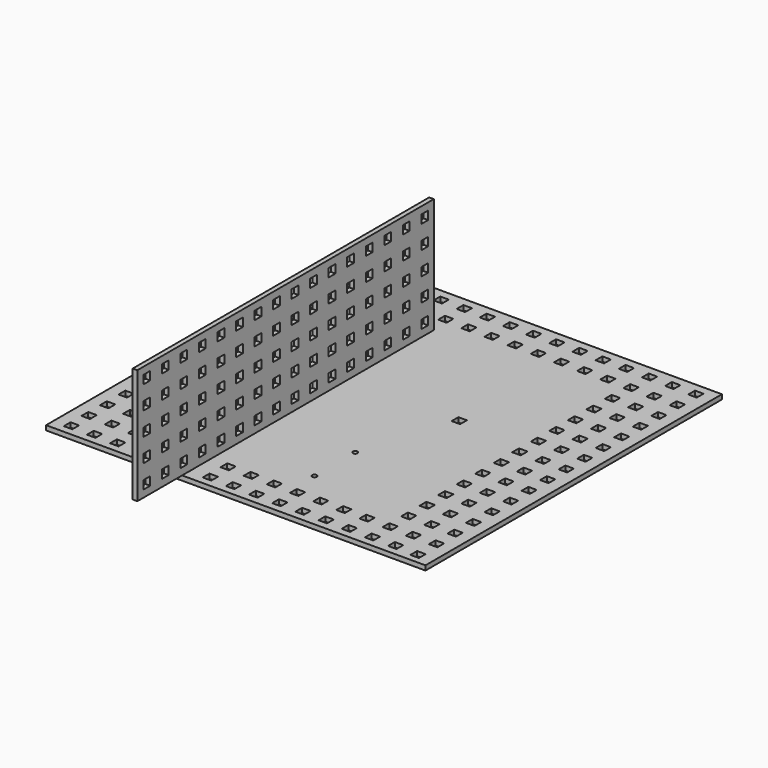
from build123d import *

# Parameters (mm, degrees)
F1_W     = 203.2
F1_H     = 63.246
F1_W_2   = 4.6228
F1_H_2   = 4.6228
F2_DEPTH = 2.54
F0_W     = 4.6482
F0_H     = 4.6228
F0_W_2   = 4.6228
F0_H_2   = 4.6482
F0_R     = 1.27
F3_DEPTH = 2.54


# Not quite as in the source:
# - a feature names something its author has since deleted; it is built from what else it names


with BuildPart() as f2:
    # F1 (on Right) → F2 (new body)
    with BuildSketch(Plane.YZ):
        with Locations((9.3608458528, 31.623)):
            Rectangle(F1_W, F1_H)
        with Locations((-85.7621541472, 6.223)):
            Rectangle(F1_W_2, F1_H_2, mode=Mode.SUBTRACT)
        with Locations((-73.0621541472, 6.223)):
            Rectangle(F1_W_2, F1_H_2, mode=Mode.SUBTRACT)
        with Locations((-60.3621541472, 6.223)):
            Rectangle(F1_W_2, F1_H_2, mode=Mode.SUBTRACT)
        with Locations((-47.6621541472, 6.223)):
            Rectangle(F1_W_2, F1_H_2, mode=Mode.SUBTRACT)
        with Locations((-34.9621541472, 6.223)):
            Rectangle(F1_W_2, F1_H_2, mode=Mode.SUBTRACT)
        with Locations((-22.2621541472, 6.223)):
            Rectangle(F1_W_2, F1_H_2, mode=Mode.SUBTRACT)
        with Locations((-9.5621541472, 6.223)):
            Rectangle(F1_W_2, F1_H_2, mode=Mode.SUBTRACT)
        with Locations((3.1378458528, 6.223)):
            Rectangle(F1_W_2, F1_H_2, mode=Mode.SUBTRACT)
        with Locations((-85.7621541472, 18.923)):
            Rectangle(F1_W_2, F1_H_2, mode=Mode.SUBTRACT)
        with Locations((-73.0621541472, 18.923)):
            Rectangle(F1_W_2, F1_H_2, mode=Mode.SUBTRACT)
        with Locations((-60.3621541472, 18.923)):
            Rectangle(F1_W_2, F1_H_2, mode=Mode.SUBTRACT)
        with Locations((-47.6621541472, 18.923)):
            Rectangle(F1_W_2, F1_H_2, mode=Mode.SUBTRACT)
        with Locations((-85.7621541472, 31.623)):
            Rectangle(F1_W_2, F1_H_2, mode=Mode.SUBTRACT)
        with Locations((-73.0621541472, 31.623)):
            Rectangle(F1_W_2, F1_H_2, mode=Mode.SUBTRACT)
        with Locations((-60.3621541472, 31.623)):
            Rectangle(F1_W_2, F1_H_2, mode=Mode.SUBTRACT)
        with Locations((-47.6621541472, 31.623)):
            Rectangle(F1_W_2, F1_H_2, mode=Mode.SUBTRACT)
        with Locations((-34.9621541472, 18.923)):
            Rectangle(F1_W_2, F1_H_2, mode=Mode.SUBTRACT)
        with Locations((-22.2621541472, 18.923)):
            Rectangle(F1_W_2, F1_H_2, mode=Mode.SUBTRACT)
        with Locations((-9.5621541472, 18.923)):
            Rectangle(F1_W_2, F1_H_2, mode=Mode.SUBTRACT)
        with Locations((3.1378458528, 18.923)):
            Rectangle(F1_W_2, F1_H_2, mode=Mode.SUBTRACT)
        with Locations((-34.9621541472, 31.623)):
            Rectangle(F1_W_2, F1_H_2, mode=Mode.SUBTRACT)
        with Locations((-22.2621541472, 31.623)):
            Rectangle(F1_W_2, F1_H_2, mode=Mode.SUBTRACT)
        with Locations((-9.5621541472, 31.623)):
            Rectangle(F1_W_2, F1_H_2, mode=Mode.SUBTRACT)
        with Locations((3.1378458528, 31.623)):
            Rectangle(F1_W_2, F1_H_2, mode=Mode.SUBTRACT)
        with Locations((15.8378458528, 6.223)):
            Rectangle(F1_W_2, F1_H_2, mode=Mode.SUBTRACT)
        with Locations((28.5378458528, 6.223)):
            Rectangle(F1_W_2, F1_H_2, mode=Mode.SUBTRACT)
        with Locations((41.2378458528, 6.223)):
            Rectangle(F1_W_2, F1_H_2, mode=Mode.SUBTRACT)
        with Locations((53.9378458528, 6.223)):
            Rectangle(F1_W_2, F1_H_2, mode=Mode.SUBTRACT)
        with Locations((66.6378458528, 6.223)):
            Rectangle(F1_W_2, F1_H_2, mode=Mode.SUBTRACT)
        with Locations((79.3378458528, 6.223)):
            Rectangle(F1_W_2, F1_H_2, mode=Mode.SUBTRACT)
        with Locations((92.0378458528, 6.223)):
            Rectangle(F1_W_2, F1_H_2, mode=Mode.SUBTRACT)
        with Locations((104.7378458528, 6.223)):
            Rectangle(F1_W_2, F1_H_2, mode=Mode.SUBTRACT)
        with Locations((15.8378458528, 18.923)):
            Rectangle(F1_W_2, F1_H_2, mode=Mode.SUBTRACT)
        with Locations((28.5378458528, 18.923)):
            Rectangle(F1_W_2, F1_H_2, mode=Mode.SUBTRACT)
        with Locations((41.2378458528, 18.923)):
            Rectangle(F1_W_2, F1_H_2, mode=Mode.SUBTRACT)
        with Locations((53.9378458528, 18.923)):
            Rectangle(F1_W_2, F1_H_2, mode=Mode.SUBTRACT)
        with Locations((15.8378458528, 31.623)):
            Rectangle(F1_W_2, F1_H_2, mode=Mode.SUBTRACT)
        with Locations((28.5378458528, 31.623)):
            Rectangle(F1_W_2, F1_H_2, mode=Mode.SUBTRACT)
        with Locations((41.2378458528, 31.623)):
            Rectangle(F1_W_2, F1_H_2, mode=Mode.SUBTRACT)
        with Locations((53.9378458528, 31.623)):
            Rectangle(F1_W_2, F1_H_2, mode=Mode.SUBTRACT)
        with Locations((66.6378458528, 18.923)):
            Rectangle(F1_W_2, F1_H_2, mode=Mode.SUBTRACT)
        with Locations((79.3378458528, 18.923)):
            Rectangle(F1_W_2, F1_H_2, mode=Mode.SUBTRACT)
        with Locations((92.0378458528, 18.923)):
            Rectangle(F1_W_2, F1_H_2, mode=Mode.SUBTRACT)
        with Locations((104.7378458528, 18.923)):
            Rectangle(F1_W_2, F1_H_2, mode=Mode.SUBTRACT)
        with Locations((66.6378458528, 31.623)):
            Rectangle(F1_W_2, F1_H_2, mode=Mode.SUBTRACT)
        with Locations((79.3378458528, 31.623)):
            Rectangle(F1_W_2, F1_H_2, mode=Mode.SUBTRACT)
        with Locations((92.0378458528, 31.623)):
            Rectangle(F1_W_2, F1_H_2, mode=Mode.SUBTRACT)
        with Locations((104.7378458528, 31.623)):
            Rectangle(F1_W_2, F1_H_2, mode=Mode.SUBTRACT)
        with Locations((-85.7621541472, 44.323)):
            Rectangle(F1_W_2, F1_H_2, mode=Mode.SUBTRACT)
        with Locations((-73.0621541472, 44.323)):
            Rectangle(F1_W_2, F1_H_2, mode=Mode.SUBTRACT)
        with Locations((-60.3621541472, 44.323)):
            Rectangle(F1_W_2, F1_H_2, mode=Mode.SUBTRACT)
        with Locations((-47.6621541472, 44.323)):
            Rectangle(F1_W_2, F1_H_2, mode=Mode.SUBTRACT)
        with Locations((-34.9621541472, 44.323)):
            Rectangle(F1_W_2, F1_H_2, mode=Mode.SUBTRACT)
        with Locations((-22.2621541472, 44.323)):
            Rectangle(F1_W_2, F1_H_2, mode=Mode.SUBTRACT)
        with Locations((-9.5621541472, 44.323)):
            Rectangle(F1_W_2, F1_H_2, mode=Mode.SUBTRACT)
        with Locations((3.1378458528, 44.323)):
            Rectangle(F1_W_2, F1_H_2, mode=Mode.SUBTRACT)
        with Locations((-85.7621541472, 57.023)):
            Rectangle(F1_W_2, F1_H_2, mode=Mode.SUBTRACT)
        with Locations((-73.0621541472, 57.023)):
            Rectangle(F1_W_2, F1_H_2, mode=Mode.SUBTRACT)
        with Locations((-60.3621541472, 57.023)):
            Rectangle(F1_W_2, F1_H_2, mode=Mode.SUBTRACT)
        with Locations((-47.6621541472, 57.023)):
            Rectangle(F1_W_2, F1_H_2, mode=Mode.SUBTRACT)
        with Locations((-34.9621541472, 57.023)):
            Rectangle(F1_W_2, F1_H_2, mode=Mode.SUBTRACT)
        with Locations((-22.2621541472, 57.023)):
            Rectangle(F1_W_2, F1_H_2, mode=Mode.SUBTRACT)
        with Locations((-9.5621541472, 57.023)):
            Rectangle(F1_W_2, F1_H_2, mode=Mode.SUBTRACT)
        with Locations((3.1378458528, 57.023)):
            Rectangle(F1_W_2, F1_H_2, mode=Mode.SUBTRACT)
        with Locations((15.8378458528, 44.323)):
            Rectangle(F1_W_2, F1_H_2, mode=Mode.SUBTRACT)
        with Locations((28.5378458528, 44.323)):
            Rectangle(F1_W_2, F1_H_2, mode=Mode.SUBTRACT)
        with Locations((41.2378458528, 44.323)):
            Rectangle(F1_W_2, F1_H_2, mode=Mode.SUBTRACT)
        with Locations((53.9378458528, 44.323)):
            Rectangle(F1_W_2, F1_H_2, mode=Mode.SUBTRACT)
        with Locations((66.6378458528, 44.323)):
            Rectangle(F1_W_2, F1_H_2, mode=Mode.SUBTRACT)
        with Locations((79.3378458528, 44.323)):
            Rectangle(F1_W_2, F1_H_2, mode=Mode.SUBTRACT)
        with Locations((92.0378458528, 44.323)):
            Rectangle(F1_W_2, F1_H_2, mode=Mode.SUBTRACT)
        with Locations((104.7378458528, 44.323)):
            Rectangle(F1_W_2, F1_H_2, mode=Mode.SUBTRACT)
        with Locations((15.8378458528, 57.023)):
            Rectangle(F1_W_2, F1_H_2, mode=Mode.SUBTRACT)
        with Locations((28.5378458528, 57.023)):
            Rectangle(F1_W_2, F1_H_2, mode=Mode.SUBTRACT)
        with Locations((41.2378458528, 57.023)):
            Rectangle(F1_W_2, F1_H_2, mode=Mode.SUBTRACT)
        with Locations((53.9378458528, 57.023)):
            Rectangle(F1_W_2, F1_H_2, mode=Mode.SUBTRACT)
        with Locations((66.6378458528, 57.023)):
            Rectangle(F1_W_2, F1_H_2, mode=Mode.SUBTRACT)
        with Locations((79.3378458528, 57.023)):
            Rectangle(F1_W_2, F1_H_2, mode=Mode.SUBTRACT)
        with Locations((92.0378458528, 57.023)):
            Rectangle(F1_W_2, F1_H_2, mode=Mode.SUBTRACT)
        with Locations((104.7378458528, 57.023)):
            Rectangle(F1_W_2, F1_H_2, mode=Mode.SUBTRACT)
    extrude(amount=F2_DEPTH)


with BuildPart() as f3:
    # F0 (on Top) → F3 (new body)
    with BuildSketch(Plane.XY):
        Polygon((136.0076294858, 98.9708560623), (136.0076294858, 111.6708560623), (136.0076294858, 124.3708560623), (136.0076294858, 141.6332916503), (-72.0437705142, 141.6332916503), (-72.0437705142, 137.0708560623), (-72.0437705142, 124.2642551661), (-72.0437705142, -40.7291439377), (-72.0437705142, -61.5667083497), (136.0076294858, -61.5667083497), (136.0076294858, -53.4291439377), (136.0076294858, -40.7291439377), (136.0076294858, -28.0291439377), (136.0076294858, -15.3291439377), (136.0076294858, -2.6291439377), (136.0076294858, 10.0708560623), (136.0076294858, 22.7708560623), (136.0076294858, 35.4708560623), (136.0076294858, 48.1708560623), (136.0076294858, 60.8708560623), (136.0076294858, 73.5708560623), (136.0076294858, 86.2708560623), align=None)
        with Locations((-63.2426705142, -55.2167083497)):
            Rectangle(F0_W, F0_H, mode=Mode.SUBTRACT)
        with Locations((-50.5426705142, -55.2167083497)):
            Rectangle(F0_W, F0_H, mode=Mode.SUBTRACT)
        Polygon((-65.5921705142, -45.3773439377), (-65.5921705142, -40.7291439377), (-65.5667705142, -40.7291439377), (-60.9439705142, -40.7291439377), (-60.9439705142, -45.3519439377), (-60.9439705142, -45.3773439377), align=None, mode=Mode.SUBTRACT)
        with Locations((-50.5553705142, -43.0405439377)):
            Rectangle(F0_W_2, F0_H, mode=Mode.SUBTRACT)
        with Locations((-37.8426705142, -55.2167083497)):
            Rectangle(F0_W, F0_H, mode=Mode.SUBTRACT)
        with Locations((-25.1426705142, -55.2167083497)):
            Rectangle(F0_W, F0_H, mode=Mode.SUBTRACT)
        with Locations((-37.8553705142, -43.0405439377)):
            Rectangle(F0_W_2, F0_H, mode=Mode.SUBTRACT)
        with Locations((-25.1553705142, -43.0405439377)):
            Rectangle(F0_W_2, F0_H, mode=Mode.SUBTRACT)
        with Locations((-63.2680705142, -30.3532439377)):
            Rectangle(F0_W, F0_H_2, mode=Mode.SUBTRACT)
        with Locations((-50.5680705142, -30.3532439377)):
            Rectangle(F0_W, F0_H_2, mode=Mode.SUBTRACT)
        with Locations((-63.2680705142, -17.6532439377)):
            Rectangle(F0_W, F0_H_2, mode=Mode.SUBTRACT)
        with Locations((-50.5680705142, -17.6532439377)):
            Rectangle(F0_W, F0_H_2, mode=Mode.SUBTRACT)
        with Locations((-37.8680705142, -30.3532439377)):
            Rectangle(F0_W, F0_H_2, mode=Mode.SUBTRACT)
        with Locations((-37.8680705142, -17.6532439377)):
            Rectangle(F0_W, F0_H_2, mode=Mode.SUBTRACT)
        with Locations((-12.4426705142, -55.2167083497)):
            Rectangle(F0_W, F0_H, mode=Mode.SUBTRACT)
        with Locations((0.2573294858, -55.2167083497)):
            Rectangle(F0_W, F0_H, mode=Mode.SUBTRACT)
        with Locations((-12.4553705142, -43.0405439377)):
            Rectangle(F0_W_2, F0_H, mode=Mode.SUBTRACT)
        with Locations((0.2446294858, -43.0405439377)):
            Rectangle(F0_W_2, F0_H, mode=Mode.SUBTRACT)
        with Locations((12.9573294858, -55.2167083497)):
            Rectangle(F0_W, F0_H, mode=Mode.SUBTRACT)
        with Locations((25.6573294858, -55.2167083497)):
            Rectangle(F0_W, F0_H, mode=Mode.SUBTRACT)
        with Locations((12.9446294858, -43.0405439377)):
            Rectangle(F0_W_2, F0_H, mode=Mode.SUBTRACT)
        with Locations((25.6446294858, -43.0405439377)):
            Rectangle(F0_W_2, F0_H, mode=Mode.SUBTRACT)
        with Locations((-4.9623705142, -34.1505439377)):
            Circle(F0_R, mode=Mode.SUBTRACT)
        with Locations((-63.2680705142, -4.9532439377)):
            Rectangle(F0_W, F0_H_2, mode=Mode.SUBTRACT)
        with Locations((-50.5680705142, -4.9532439377)):
            Rectangle(F0_W, F0_H_2, mode=Mode.SUBTRACT)
        with Locations((-63.2680705142, 7.7467560623)):
            Rectangle(F0_W, F0_H_2, mode=Mode.SUBTRACT)
        with Locations((-50.5680705142, 7.7467560623)):
            Rectangle(F0_W, F0_H_2, mode=Mode.SUBTRACT)
        with Locations((-37.8680705142, -4.9532439377)):
            Rectangle(F0_W, F0_H_2, mode=Mode.SUBTRACT)
        with Locations((-37.8680705142, 7.7467560623)):
            Rectangle(F0_W, F0_H_2, mode=Mode.SUBTRACT)
        with Locations((-63.2680705142, 20.4467560623)):
            Rectangle(F0_W, F0_H_2, mode=Mode.SUBTRACT)
        with Locations((-50.5680705142, 20.4467560623)):
            Rectangle(F0_W, F0_H_2, mode=Mode.SUBTRACT)
        with Locations((-63.2680705142, 33.1467560623)):
            Rectangle(F0_W, F0_H_2, mode=Mode.SUBTRACT)
        with Locations((-50.5680705142, 33.1467560623)):
            Rectangle(F0_W, F0_H_2, mode=Mode.SUBTRACT)
        with Locations((-37.8680705142, 20.4467560623)):
            Rectangle(F0_W, F0_H_2, mode=Mode.SUBTRACT)
        with Locations((-37.8680705142, 33.1467560623)):
            Rectangle(F0_W, F0_H_2, mode=Mode.SUBTRACT)
        with Locations((-3.6923705142, 14.1094560623)):
            Circle(F0_R, mode=Mode.SUBTRACT)
        with Locations((38.3573294858, -55.2167083497)):
            Rectangle(F0_W, F0_H, mode=Mode.SUBTRACT)
        with Locations((51.0573294858, -55.2167083497)):
            Rectangle(F0_W, F0_H, mode=Mode.SUBTRACT)
        with Locations((38.3446294858, -43.0405439377)):
            Rectangle(F0_W_2, F0_H, mode=Mode.SUBTRACT)
        with Locations((51.0446294858, -43.0405439377)):
            Rectangle(F0_W_2, F0_H, mode=Mode.SUBTRACT)
        with Locations((63.7573294858, -55.2167083497)):
            Rectangle(F0_W, F0_H, mode=Mode.SUBTRACT)
        with Locations((76.4573294858, -55.2167083497)):
            Rectangle(F0_W, F0_H, mode=Mode.SUBTRACT)
        with Locations((63.7446294858, -43.0405439377)):
            Rectangle(F0_W_2, F0_H, mode=Mode.SUBTRACT)
        with Locations((76.4446294858, -43.0405439377)):
            Rectangle(F0_W_2, F0_H, mode=Mode.SUBTRACT)
        with Locations((47.1076294858, -26.5305439377)):
            Circle(F0_R, mode=Mode.SUBTRACT)
        with Locations((89.1573294858, -55.2167083497)):
            Rectangle(F0_W, F0_H, mode=Mode.SUBTRACT)
        with Locations((101.8573294858, -55.2167083497)):
            Rectangle(F0_W, F0_H, mode=Mode.SUBTRACT)
        with Locations((89.1446294858, -43.0405439377)):
            Rectangle(F0_W_2, F0_H, mode=Mode.SUBTRACT)
        with Locations((101.8446294858, -43.0405439377)):
            Rectangle(F0_W_2, F0_H, mode=Mode.SUBTRACT)
        with Locations((114.5573294858, -55.2167083497)):
            Rectangle(F0_W, F0_H, mode=Mode.SUBTRACT)
        with Locations((127.2446294858, -55.7405439377)):
            Rectangle(F0_W_2, F0_H, mode=Mode.SUBTRACT)
        with Locations((114.5446294858, -43.0405439377)):
            Rectangle(F0_W_2, F0_H, mode=Mode.SUBTRACT)
        with Locations((127.2446294858, -43.0405439377)):
            Rectangle(F0_W_2, F0_H, mode=Mode.SUBTRACT)
        with Locations((101.8319294858, -30.3532439377)):
            Rectangle(F0_W, F0_H_2, mode=Mode.SUBTRACT)
        with Locations((101.8319294858, -17.6532439377)):
            Rectangle(F0_W, F0_H_2, mode=Mode.SUBTRACT)
        with Locations((114.5319294858, -30.3405439377)):
            Rectangle(F0_W, F0_H, mode=Mode.SUBTRACT)
        with Locations((127.2446294858, -30.3405439377)):
            Rectangle(F0_W_2, F0_H, mode=Mode.SUBTRACT)
        with Locations((114.5319294858, -17.6405439377)):
            Rectangle(F0_W, F0_H, mode=Mode.SUBTRACT)
        with Locations((127.2446294858, -17.6405439377)):
            Rectangle(F0_W_2, F0_H, mode=Mode.SUBTRACT)
        with Locations((47.1076294858, 1.4094560623)):
            Circle(F0_R, mode=Mode.SUBTRACT)
        with Locations((101.8319294858, -4.9532439377)):
            Rectangle(F0_W, F0_H_2, mode=Mode.SUBTRACT)
        with Locations((101.8319294858, 7.7467560623)):
            Rectangle(F0_W, F0_H_2, mode=Mode.SUBTRACT)
        with Locations((114.5319294858, -4.9405439377)):
            Rectangle(F0_W, F0_H, mode=Mode.SUBTRACT)
        with Locations((127.2446294858, -4.9405439377)):
            Rectangle(F0_W_2, F0_H, mode=Mode.SUBTRACT)
        with Locations((114.5319294858, 7.7594560623)):
            Rectangle(F0_W, F0_H, mode=Mode.SUBTRACT)
        with Locations((127.2446294858, 7.7594560623)):
            Rectangle(F0_W_2, F0_H, mode=Mode.SUBTRACT)
        with Locations((101.8319294858, 20.4467560623)):
            Rectangle(F0_W, F0_H_2, mode=Mode.SUBTRACT)
        with Locations((101.8319294858, 33.1467560623)):
            Rectangle(F0_W, F0_H_2, mode=Mode.SUBTRACT)
        with Locations((114.5319294858, 20.4594560623)):
            Rectangle(F0_W, F0_H, mode=Mode.SUBTRACT)
        with Locations((127.2446294858, 20.4594560623)):
            Rectangle(F0_W_2, F0_H, mode=Mode.SUBTRACT)
        with Locations((114.5319294858, 33.1594560623)):
            Rectangle(F0_W, F0_H, mode=Mode.SUBTRACT)
        with Locations((127.2446294858, 33.1594560623)):
            Rectangle(F0_W_2, F0_H, mode=Mode.SUBTRACT)
        with Locations((-63.2680705142, 45.8467560623)):
            Rectangle(F0_W, F0_H_2, mode=Mode.SUBTRACT)
        with Locations((-50.5680705142, 45.8467560623)):
            Rectangle(F0_W, F0_H_2, mode=Mode.SUBTRACT)
        with Locations((-63.2680705142, 58.5467560623)):
            Rectangle(F0_W, F0_H_2, mode=Mode.SUBTRACT)
        with Locations((-50.5680705142, 58.5467560623)):
            Rectangle(F0_W, F0_H_2, mode=Mode.SUBTRACT)
        with Locations((-37.8680705142, 45.8467560623)):
            Rectangle(F0_W, F0_H_2, mode=Mode.SUBTRACT)
        with Locations((-37.8680705142, 58.5467560623)):
            Rectangle(F0_W, F0_H_2, mode=Mode.SUBTRACT)
        with Locations((-63.2680705142, 71.2467560623)):
            Rectangle(F0_W, F0_H_2, mode=Mode.SUBTRACT)
        with Locations((-50.5680705142, 71.2467560623)):
            Rectangle(F0_W, F0_H_2, mode=Mode.SUBTRACT)
        with Locations((-63.2680705142, 83.9467560623)):
            Rectangle(F0_W, F0_H_2, mode=Mode.SUBTRACT)
        with Locations((-50.5680705142, 83.9467560623)):
            Rectangle(F0_W, F0_H_2, mode=Mode.SUBTRACT)
        with Locations((-37.8680705142, 71.2467560623)):
            Rectangle(F0_W, F0_H_2, mode=Mode.SUBTRACT)
        with Locations((-37.8680705142, 83.9467560623)):
            Rectangle(F0_W, F0_H_2, mode=Mode.SUBTRACT)
        with Locations((0, 52.209622947)):
            Rectangle(F0_W, F0_H_2, mode=Mode.SUBTRACT)
        with Locations((-63.2680705142, 96.6467560623)):
            Rectangle(F0_W, F0_H_2, mode=Mode.SUBTRACT)
        with Locations((-50.5680705142, 96.6467560623)):
            Rectangle(F0_W, F0_H_2, mode=Mode.SUBTRACT)
        with Locations((-63.2680705142, 109.3467560623)):
            Rectangle(F0_W, F0_H_2, mode=Mode.SUBTRACT)
        with Locations((-50.5680705142, 109.3467560623)):
            Rectangle(F0_W, F0_H_2, mode=Mode.SUBTRACT)
        with Locations((-37.8680705142, 96.6467560623)):
            Rectangle(F0_W, F0_H_2, mode=Mode.SUBTRACT)
        with Locations((-37.8680705142, 109.3467560623)):
            Rectangle(F0_W, F0_H_2, mode=Mode.SUBTRACT)
        Polygon((-65.5921705142, 119.7226560623), (-65.5921705142, 124.2642551661), (-65.5921705142, 124.3708560623), (-60.9439705142, 124.3708560623), (-60.9439705142, 119.7226560623), align=None, mode=Mode.SUBTRACT)
        with Locations((-50.5680705142, 122.0467560623)):
            Rectangle(F0_W, F0_H_2, mode=Mode.SUBTRACT)
        with Locations((-63.2680705142, 134.7467560623)):
            Rectangle(F0_W, F0_H_2, mode=Mode.SUBTRACT)
        with Locations((-50.5680705142, 134.7467560623)):
            Rectangle(F0_W, F0_H_2, mode=Mode.SUBTRACT)
        with Locations((-37.8680705142, 122.0467560623)):
            Rectangle(F0_W, F0_H_2, mode=Mode.SUBTRACT)
        with Locations((-25.1680705142, 122.0467560623)):
            Rectangle(F0_W, F0_H_2, mode=Mode.SUBTRACT)
        with Locations((-37.8680705142, 134.7467560623)):
            Rectangle(F0_W, F0_H_2, mode=Mode.SUBTRACT)
        with Locations((-25.1680705142, 134.7467560623)):
            Rectangle(F0_W, F0_H_2, mode=Mode.SUBTRACT)
        with Locations((-12.4680705142, 122.0467560623)):
            Rectangle(F0_W, F0_H_2, mode=Mode.SUBTRACT)
        with Locations((0.2319294858, 122.0467560623)):
            Rectangle(F0_W, F0_H_2, mode=Mode.SUBTRACT)
        with Locations((-12.4680705142, 134.7467560623)):
            Rectangle(F0_W, F0_H_2, mode=Mode.SUBTRACT)
        with Locations((0.2319294858, 134.7467560623)):
            Rectangle(F0_W, F0_H_2, mode=Mode.SUBTRACT)
        with Locations((12.9319294858, 122.0467560623)):
            Rectangle(F0_W, F0_H_2, mode=Mode.SUBTRACT)
        with Locations((25.6319294858, 122.0467560623)):
            Rectangle(F0_W, F0_H_2, mode=Mode.SUBTRACT)
        with Locations((12.9319294858, 134.7467560623)):
            Rectangle(F0_W, F0_H_2, mode=Mode.SUBTRACT)
        with Locations((25.6319294858, 134.7467560623)):
            Rectangle(F0_W, F0_H_2, mode=Mode.SUBTRACT)
        with Locations((63.5, 52.209622947)):
            Rectangle(F0_W, F0_H_2, mode=Mode.SUBTRACT)
        with Locations((101.8319294858, 45.8467560623)):
            Rectangle(F0_W, F0_H_2, mode=Mode.SUBTRACT)
        with Locations((101.8319294858, 58.5467560623)):
            Rectangle(F0_W, F0_H_2, mode=Mode.SUBTRACT)
        with Locations((114.5319294858, 45.8594560623)):
            Rectangle(F0_W, F0_H, mode=Mode.SUBTRACT)
        with Locations((127.2446294858, 45.8594560623)):
            Rectangle(F0_W_2, F0_H, mode=Mode.SUBTRACT)
        with Locations((114.5319294858, 58.5594560623)):
            Rectangle(F0_W, F0_H, mode=Mode.SUBTRACT)
        with Locations((127.2446294858, 58.5594560623)):
            Rectangle(F0_W_2, F0_H, mode=Mode.SUBTRACT)
        with Locations((101.8319294858, 71.2467560623)):
            Rectangle(F0_W, F0_H_2, mode=Mode.SUBTRACT)
        with Locations((101.8319294858, 83.9467560623)):
            Rectangle(F0_W, F0_H_2, mode=Mode.SUBTRACT)
        with Locations((114.5319294858, 71.2594560623)):
            Rectangle(F0_W, F0_H, mode=Mode.SUBTRACT)
        with Locations((127.2446294858, 71.2594560623)):
            Rectangle(F0_W_2, F0_H, mode=Mode.SUBTRACT)
        with Locations((114.5319294858, 83.9594560623)):
            Rectangle(F0_W, F0_H, mode=Mode.SUBTRACT)
        with Locations((127.2446294858, 83.9594560623)):
            Rectangle(F0_W_2, F0_H, mode=Mode.SUBTRACT)
        with Locations((38.3319294858, 122.0467560623)):
            Rectangle(F0_W, F0_H_2, mode=Mode.SUBTRACT)
        with Locations((51.0319294858, 122.0467560623)):
            Rectangle(F0_W, F0_H_2, mode=Mode.SUBTRACT)
        with Locations((38.3319294858, 134.7467560623)):
            Rectangle(F0_W, F0_H_2, mode=Mode.SUBTRACT)
        with Locations((51.0319294858, 134.7467560623)):
            Rectangle(F0_W, F0_H_2, mode=Mode.SUBTRACT)
        with Locations((63.7319294858, 122.0467560623)):
            Rectangle(F0_W, F0_H_2, mode=Mode.SUBTRACT)
        with Locations((76.4319294858, 122.0467560623)):
            Rectangle(F0_W, F0_H_2, mode=Mode.SUBTRACT)
        with Locations((63.7319294858, 134.7467560623)):
            Rectangle(F0_W, F0_H_2, mode=Mode.SUBTRACT)
        with Locations((76.4319294858, 134.7467560623)):
            Rectangle(F0_W, F0_H_2, mode=Mode.SUBTRACT)
        with Locations((101.8319294858, 96.6467560623)):
            Rectangle(F0_W, F0_H_2, mode=Mode.SUBTRACT)
        with Locations((101.8319294858, 109.3467560623)):
            Rectangle(F0_W, F0_H_2, mode=Mode.SUBTRACT)
        with Locations((114.5319294858, 96.6594560623)):
            Rectangle(F0_W, F0_H, mode=Mode.SUBTRACT)
        with Locations((127.2446294858, 96.6594560623)):
            Rectangle(F0_W_2, F0_H, mode=Mode.SUBTRACT)
        with Locations((114.5319294858, 109.3594560623)):
            Rectangle(F0_W, F0_H, mode=Mode.SUBTRACT)
        with Locations((127.2319294858, 109.3594560623)):
            Rectangle(F0_W, F0_H, mode=Mode.SUBTRACT)
        with Locations((89.1319294858, 122.0467560623)):
            Rectangle(F0_W, F0_H_2, mode=Mode.SUBTRACT)
        with Locations((101.8319294858, 122.0467560623)):
            Rectangle(F0_W, F0_H_2, mode=Mode.SUBTRACT)
        with Locations((89.1319294858, 134.7467560623)):
            Rectangle(F0_W, F0_H_2, mode=Mode.SUBTRACT)
        with Locations((101.8319294858, 134.7467560623)):
            Rectangle(F0_W, F0_H_2, mode=Mode.SUBTRACT)
        with Locations((114.5319294858, 122.0467560623)):
            Rectangle(F0_W, F0_H_2, mode=Mode.SUBTRACT)
        with Locations((127.2319294858, 122.0467560623)):
            Rectangle(F0_W, F0_H_2, mode=Mode.SUBTRACT)
        with Locations((114.5319294858, 134.7467560623)):
            Rectangle(F0_W, F0_H_2, mode=Mode.SUBTRACT)
        with Locations((127.2319294858, 134.7467560623)):
            Rectangle(F0_W, F0_H_2, mode=Mode.SUBTRACT)
    extrude(amount=-F3_DEPTH)


solid = Compound([f2.part, f3.part])
